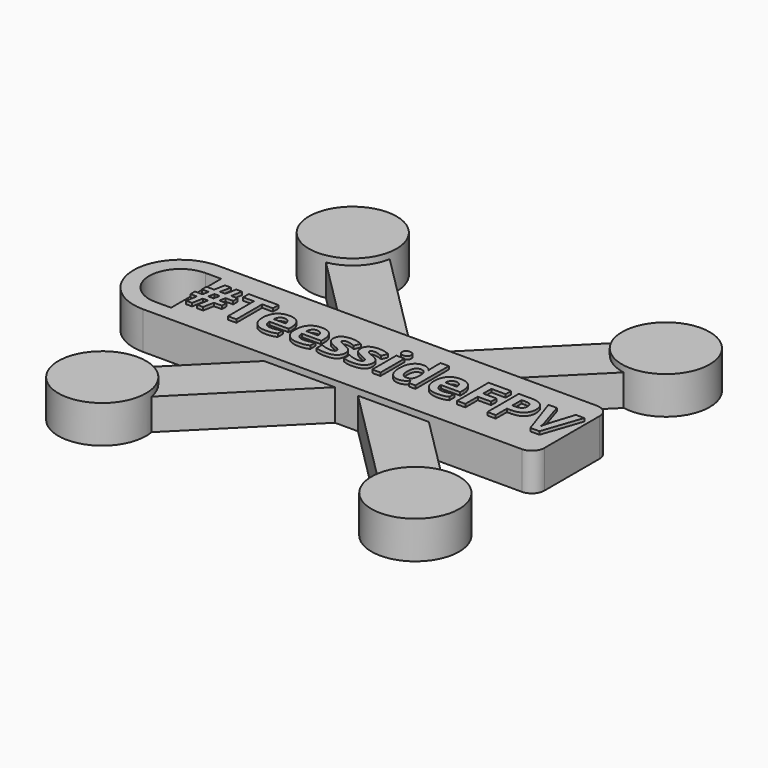
from build123d import *

# Parameters (mm, degrees)
F1_W         = 30
F1_H         = 7.5
F2_DEPTH     = 3
F1_R         = 3.5
F3_TEXT_SIZE = 4.3982223851
F4_DEPTH     = 0.25
F6_DEPTH     = 2.5
F7_DEPTH     = 5
F8_R         = 3.74999
F10_DEPTH    = 25
F11_R        = 1


# Not quite as in the source:
# - a fillet or chamfer is up to 0.001 mm smaller than in the source, because OpenCascade refuses the exact size
# - Text() gives the source's letters only with a copy of the font that has no kerning and outlines rounded to 1/6400 em; it was checked with that copy


with BuildPart() as f2:
    # F1 (on Top) → F2 (new body)
    with BuildSketch(Plane.XY):
        Rectangle(F1_W, F1_H)
    extrude(amount=F2_DEPTH)



with BuildPart() as f2b:
    # F1 (on Top) → F2, piece 2 (new body)
    with BuildSketch(Plane.XY):
        with Locations((-12.5, 12.5)):
            Circle(F1_R)
    extrude(amount=F2_DEPTH)


with BuildPart() as f2c:
    # F1 (on Top) → F2, piece 3 (new body)
    with BuildSketch(Plane.XY):
        with Locations((-12.5, -12.5)):
            Circle(F1_R)
    extrude(amount=F2_DEPTH)


with BuildPart() as f2d:
    # F1 (on Top) → F2, piece 4 (new body)
    with BuildSketch(Plane.XY):
        with Locations((12.5, -12.5)):
            Circle(F1_R)
    extrude(amount=F2_DEPTH)


with BuildPart() as f2e:
    # F1 (on Top) → F2, piece 5 (new body)
    with BuildSketch(Plane.XY):
        with Locations((12.5, 12.5)):
            Circle(F1_R)
    extrude(amount=F2_DEPTH)


with BuildPart() as f4:
    # F3 (on face) → F4 (new body, symmetric)
    with BuildSketch(Plane.XY.offset(3)):
        with Locations((-15, -1.5522687726)):
            Text('#TeessideFPV', F3_TEXT_SIZE, font='Open Sans', font_style=FontStyle.BOLD, text_align=(TextAlign.LEFT, TextAlign.BOTTOM))
    extrude(amount=F4_DEPTH, both=True)


with BuildPart() as f2_1:
    add(f2.part)

    add(f2b.part)  # F6 merges F2b

    add(f2c.part)  # F6 merges F2c

    add(f2d.part)  # F6 merges F2d

    add(f2e.part)  # F6 merges F2e
    # F5 (on face) → F6 (join)
    with BuildSketch(Plane(origin=(0, 0, 0), x_dir=(1, 0, 0), z_dir=(0, 0, -1))):
        Polygon((13.9142135624, 11.0857864376), (11.0857864376, 13.9142135624), (0, 2.8284271247), (2.8284271247, 0), align=None)
        Polygon((2.8284271247, 0), (0, 2.8284271247), (-2.8284271247, 0), (0, -2.8284271247), align=None)
        Polygon((-2.8284271247, 0), (0, 2.8284271247), (-11.0857864376, 13.9142135624), (-13.9142135624, 11.0857864376), align=None)
        Polygon((0, -2.8284271247), (-2.8284271247, 0), (-13.9142135624, -11.0857864376), (-11.0857864376, -13.9142135624), align=None)
        Polygon((13.9142135624, -11.0857864376), (2.8284271247, 0), (0, -2.8284271247), (11.0857864376, -13.9142135624), align=None)
    extrude(amount=-F6_DEPTH)

    # F7 (add): a face of the model
    f7_faces = [f2_1.faces().sort_by_distance(p)[0] for p in [
        (-15, 0, 1.5),
    ]]
    extrude(f7_faces, amount=F7_DEPTH)

    # F8 (radius 3.75 in the source; OpenCascade refuses exactly that, so slightly less here)
    f8_edges = [f2_1.edges().sort_by_distance(p)[0] for p in [
        (-20, 3.75, 1.5),
        (-20, -3.75, 1.5),
    ]]
    fillet(f8_edges, radius=F8_R)

    # F9 (on face) → F10 (cut)
    with BuildSketch(Plane.XY.offset(3)):
        with BuildLine():
            Line((-15, 2.5), (-16.25, 2.5))
            ThreePointArc((-16.25, 2.5), (-18.75, 0), (-16.25, -2.5))
            Line((-16.25, -2.5), (-15, -2.5))
            Line((-15, -2.5), (-15, 2.5))
        make_face()
    extrude(amount=-F10_DEPTH, mode=Mode.SUBTRACT)

    # F11
    f11_edges = [f2_1.edges().sort_by_distance(p)[0] for p in [
        (15, -3.75, 1.5),
        (15, 3.75, 1.5),
    ]]
    fillet(f11_edges, radius=F11_R)


solid = Compound([f4.part, f2_1.part])
